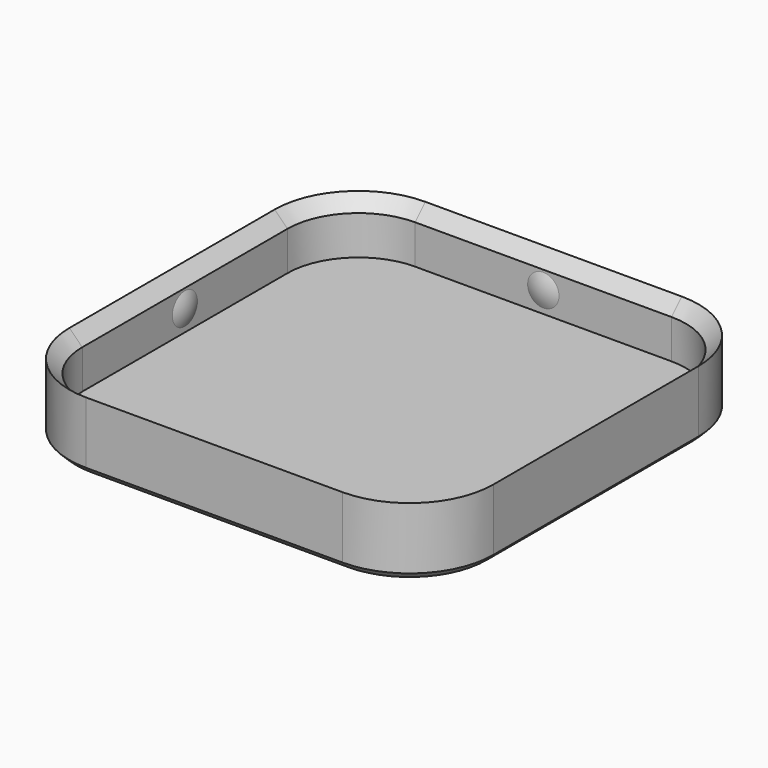
from build123d import *

# Parameters (mm, degrees)
F1_DEPTH        = 4.65
F0_R            = 5.153196002
F2_DEPTH        = 1.5
F3_SIZE         = 1.14999
F4_SIZE         = 0.6
F7_ANGLE        = 180
F8_DEPTH        = 1.5
F9_COUNT        = 4
F10_W           = 35
F10_H           = 1
F10_TEXT_SIZE   = 7.064234248
F10_TEXT_SIZE_2 = 8.7888613389
F11_DEPTH       = 0.4


# Not quite as in the source:
# - a fillet or chamfer is up to 0.001 mm smaller than in the source, because OpenCascade refuses the exact size
# - Text() gives the source's letters only with a copy of the font that has no kerning and outlines rounded to 1/6400 em; it was checked with that copy


with BuildPart() as f1:
    # F0 (on Top) → F1 (new body)
    with BuildSketch(Plane.XY):
        with BuildLine():
            ThreePointArc((19, 11.5), (16.8033008589, 16.8033008589), (11.5, 19))
            Line((11.5, 19), (-11.5, 19))
            ThreePointArc((-11.5, 19), (-16.8033008589, 16.8033008589), (-19, 11.5))
            Line((-19, 11.5), (-19, -11.5))
            ThreePointArc((-19, -11.5), (-16.8033008589, -16.8033008589), (-11.5, -19))
            Line((-11.5, -19), (11.5, -19))
            ThreePointArc((11.5, -19), (16.8033008589, -16.8033008589), (19, -11.5))
            Line((19, -11.5), (19, 11.5))
        make_face()
        with BuildLine():
            Line((-11.5, 17.85), (11.5, 17.85))
            ThreePointArc((11.5, 17.85), (15.9901280605, 15.9901280605), (17.85, 11.5))
            Line((17.85, 11.5), (17.85, -11.5))
            ThreePointArc((17.85, -11.5), (15.9901280605, -15.9901280605), (11.5, -17.85))
            Line((11.5, -17.85), (-11.5, -17.85))
            ThreePointArc((-11.5, -17.85), (-15.9901280605, -15.9901280605), (-17.85, -11.5))
            Line((-17.85, -11.5), (-17.85, 11.5))
            ThreePointArc((-17.85, 11.5), (-15.9901280605, 15.9901280605), (-11.5, 17.85))
        make_face(mode=Mode.SUBTRACT)
    extrude(amount=F1_DEPTH)

    # F0 (on Top) → F2 (join)
    with BuildSketch(Plane.XY):
        with BuildLine():
            ThreePointArc((19, 11.5), (16.8033008589, 16.8033008589), (11.5, 19))
            Line((11.5, 19), (-11.5, 19))
            ThreePointArc((-11.5, 19), (-16.8033008589, 16.8033008589), (-19, 11.5))
            Line((-19, 11.5), (-19, -11.5))
            ThreePointArc((-19, -11.5), (-16.8033008589, -16.8033008589), (-11.5, -19))
            Line((-11.5, -19), (11.5, -19))
            ThreePointArc((11.5, -19), (16.8033008589, -16.8033008589), (19, -11.5))
            Line((19, -11.5), (19, 11.5))
        make_face()
        with BuildLine():
            Line((-11.5, 17.85), (11.5, 17.85))
            ThreePointArc((11.5, 17.85), (15.9901280605, 15.9901280605), (17.85, 11.5))
            Line((17.85, 11.5), (17.85, -11.5))
            ThreePointArc((17.85, -11.5), (15.9901280605, -15.9901280605), (11.5, -17.85))
            Line((11.5, -17.85), (-11.5, -17.85))
            ThreePointArc((-11.5, -17.85), (-15.9901280605, -15.9901280605), (-17.85, -11.5))
            Line((-17.85, -11.5), (-17.85, 11.5))
            ThreePointArc((-17.85, 11.5), (-15.9901280605, 15.9901280605), (-11.5, 17.85))
        make_face(mode=Mode.SUBTRACT)
        with BuildLine():
            ThreePointArc((17.85, 11.5), (15.9901280605, 15.9901280605), (11.5, 17.85))
            Line((11.5, 17.85), (-11.5, 17.85))
            ThreePointArc((-11.5, 17.85), (-15.9901280605, 15.9901280605), (-17.85, 11.5))
            Line((-17.85, 11.5), (-17.85, -11.5))
            ThreePointArc((-17.85, -11.5), (-15.9901280605, -15.9901280605), (-11.5, -17.85))
            Line((-11.5, -17.85), (11.5, -17.85))
            ThreePointArc((11.5, -17.85), (15.9901280605, -15.9901280605), (17.85, -11.5))
            Line((17.85, -11.5), (17.85, 11.5))
        make_face()
        Circle(F0_R, mode=Mode.SUBTRACT)
        Circle(F0_R)
    extrude(amount=-F2_DEPTH)

    # F3 (size 1.15 in the source; OpenCascade refuses exactly that, so slightly less here)
    f3_edges = [f1.edges().sort_by_distance(p)[0] for p in [
        (-17.85, 0, 4.65),
    ]]
    chamfer(f3_edges, length=F3_SIZE)

    # F4
    f4_edges = [f1.edges().sort_by_distance(p)[0] for p in [
        (19, 0, -1.5),
        (16.803301, 16.803301, -1.5),
        (0, 19, -1.5),
        (-16.803301, 16.803301, -1.5),
        (-19, 0, -1.5),
        (-16.803301, -16.803301, -1.5),
        (0, -19, -1.5),
        (16.803301, -16.803301, -1.5),
    ]]
    chamfer(f4_edges, length=F4_SIZE)

    # F6 (on offset) → F7 (revolve)
    with BuildSketch(Plane.XZ.offset(20.5)):
        with BuildLine():
            Line((0, 4.875), (0, -1.125))
            ThreePointArc((0, -1.125), (3, 1.875), (0, 4.875))
        make_face()
    revolve(axis=Axis((0, -20.5, 1.875), (0, 0, 1)), revolution_arc=F7_ANGLE)

    # F8 (cut, through all): a face of the model
    f8_faces = [f1.faces().sort_by_distance(p)[0] for p in [
        (0, -20.5, 1.875),
    ]]
    extrude(f8_faces, amount=-F8_DEPTH, mode=Mode.SUBTRACT)

    # F9: F1 ×4 about axis
    f9_axis = Axis((0, 0, 0), (0, 0, 1))


with BuildPart() as f1_1:
    add(f1.part)
    for i in range(1, F9_COUNT):
        add(f1.part.rotate(f9_axis, i * 360 / F9_COUNT))

    # F10 (on face) → F11 (cut)
    with BuildSketch(Plane(origin=(0, 0, -1.5), x_dir=(1, 0, 0), z_dir=(0, 0, -1))):
        with Locations((0, 0.5261319457)):
            Rectangle(F10_W, F10_H)
        with Locations((-18, 2.8122555413)):
            Text('RUNCAM3', F10_TEXT_SIZE, font='Open Sans', font_style=FontStyle.BOLD, text_align=(TextAlign.LEFT, TextAlign.BOTTOM))
        with Locations((-17.4814747043, -8.0791096006)):
            Text('AIRSTER', F10_TEXT_SIZE_2, font='Open Sans', font_style=FontStyle.BOLD, text_align=(TextAlign.LEFT, TextAlign.BOTTOM))
    extrude(amount=-F11_DEPTH, mode=Mode.SUBTRACT)


solid = f1_1.part
